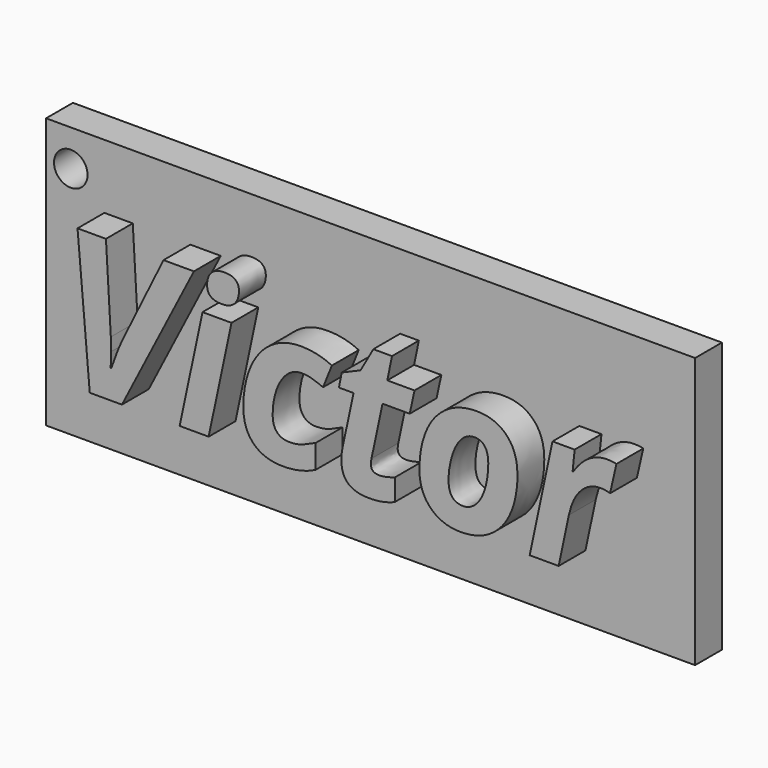
from build123d import *

# Parameters (mm, degrees)
F0_W         = 122.8719390929
F0_H         = 51.1966440827
F1_DEPTH     = 6.35
F2_TEXT_SIZE = 37.3308844347
F3_DEPTH     = 6.35
F5_D         = 6.35


# Not quite as in the source:
# - Text() gives the source's letters only with a copy of the font that has no kerning and outlines rounded to 1/6400 em; it was checked with that copy


with BuildPart() as f1:
    # F0 (on Front) → F1 (new body)
    with BuildSketch(Plane.XZ):
        with Locations((3.6264266819, 2.986474894)):
            Rectangle(F0_W, F0_H)
    extrude(amount=F1_DEPTH)

    # F2 (on face) → F3 (join)
    with BuildSketch(Plane.XZ.offset(6.35)):
        with Locations((-50.1300469041, -10.2393245324)):
            Text('Victor', F2_TEXT_SIZE, font='Open Sans', font_style=FontStyle.BOLDITALIC, text_align=(TextAlign.LEFT, TextAlign.BOTTOM))
    extrude(amount=F3_DEPTH)

    # F5 (through all)
    with Locations(Plane.XZ.offset(6.35)):
        with Locations((-53.1350411475, 21.7020679265)):
            Hole(F5_D / 2)


solid = f1.part
